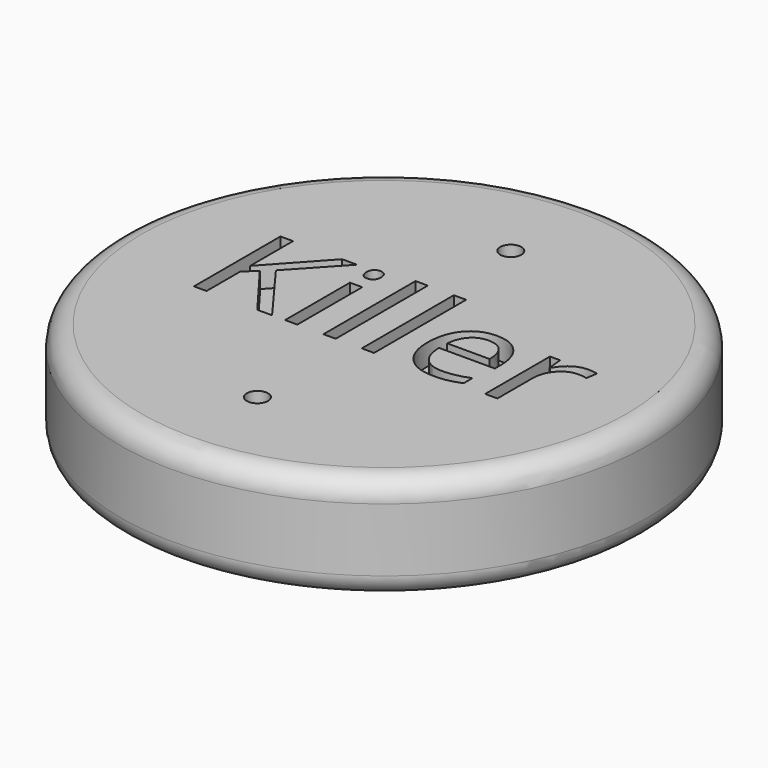
from build123d import *

# Parameters (mm, degrees)
F0_R           = 25
F1_DEPTH       = 10
F2_R           = 2
F4_D           = 2
F4_CBORE_D     = 5
F4_CBORE_DEPTH = 2.5
F5_TEXT_SIZE   = 14.3517895291
F6_DEPTH       = 2


# Not quite as in the source:
# - Text() gives the source's letters only with a copy of the font that has no kerning and outlines rounded to 1/6400 em; it was checked with that copy


with BuildPart() as f1:
    # F0 (on Top) → F1 (new body)
    with BuildSketch(Plane.XY):
        Circle(F0_R)
    extrude(amount=F1_DEPTH)

    # F2
    f2_edges = [f1.edges().sort_by_distance(p)[0] for p in [
        (-25, 0, 10),
        (-25, 0, 0),
    ]]
    fillet(f2_edges, radius=F2_R)

    # F4 (through all)
    with Locations(Plane(origin=(0, 0, 0), x_dir=(1, 0, 0), z_dir=(0, 0, -1))):
        with Locations((0, 15), (0, -15)):
            CounterBoreHole(F4_D / 2, F4_CBORE_D / 2, F4_CBORE_DEPTH)

    # F5 (on face) → F6 (cut)
    with BuildSketch(Plane.XY.offset(10)):
        with Locations((-16.1527623422, -4.0809251659)):
            Text('Killer', F5_TEXT_SIZE, font='Open Sans', text_align=(TextAlign.LEFT, TextAlign.BOTTOM))
    extrude(amount=-F6_DEPTH, mode=Mode.SUBTRACT)


solid = f1.part
